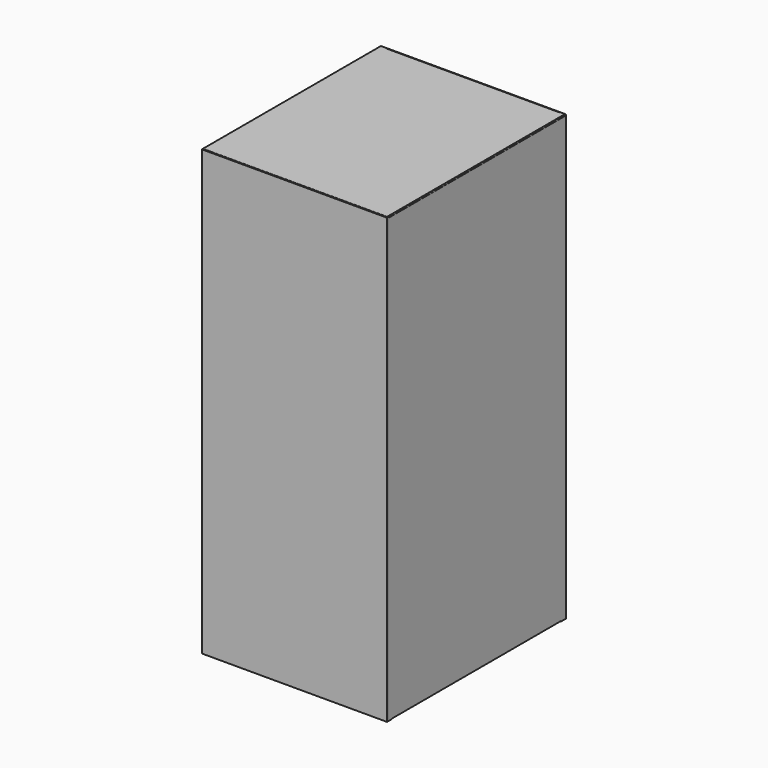
from build123d import *

# Parameters (mm, degrees)
F1_DEPTH       = 914.4
F3_DEPTH       = 1828.8
F5_DEPTH       = 749.3
F6_R           = 6.35
F6_W           = 3.175
F6_H           = 487.3625
F6_H_2         = 6.35
F6_H_3         = 31.75
F7_DEPTH       = 50.8
F7_DEPTH_BACK  = 50.8
F8_W           = 850.9
F8_H           = 1111.25
F9_DEPTH       = 1.016
F10_W          = 3.175
F10_H          = 25.4
F11_DEPTH      = 581.026
F11_DEPTH_BACK = 180.976
F13_W          = 850.9
F13_H          = 1111.25
F14_DEPTH      = 1.016
F12_W          = 914.4
F12_H          = 1823.2365249493
F16_DEPTH      = 0.8128
F15_W          = 920.75
F15_H          = 1828.8
F17_DEPTH      = 0.8128
F18_W          = 758.825
F18_H          = 914.4
F19_DEPTH      = 0.8128
F20_W          = 755.65
F20_H          = 914.4
F21_DEPTH      = 0.8128
F22_W          = 755.65
F22_H          = 1828.8
F23_DEPTH      = 0.8128
F24_W          = 762
F24_H          = 1828.8
F25_DEPTH      = 0.8128


with BuildPart() as f1:
    # F0 (on Front) → F1 (new body)
    with BuildSketch(Plane.XZ):
        Polygon((0, 25.4), (0, 0), (25.4, 0), (25.4, 3.175), (3.175, 3.175), (3.175, 25.4), align=None)
    extrude(amount=-F1_DEPTH)


with BuildPart() as f1b:
    # F0 (on Front) → F1, piece 2 (new body)
    with BuildSketch(Plane.XZ):
        Polygon((730.25, 3.175), (730.25, 0), (755.65, 0), (755.65, 25.4), (752.475, 25.4), (752.475, 3.175), align=None)
    extrude(amount=-F1_DEPTH)


with BuildPart() as f1c:
    # F0 (on Front) → F1, piece 3 (new body)
    with BuildSketch(Plane.XZ):
        Polygon((755.65, 1828.8), (730.25, 1828.8), (730.25, 1825.625), (752.475, 1825.625), (752.475, 1803.4), (755.65, 1803.4), align=None)
    extrude(amount=-F1_DEPTH)


with BuildPart() as f1d:
    # F0 (on Front) → F1, piece 4 (new body)
    with BuildSketch(Plane.XZ):
        Polygon((0, 1828.8), (0, 1803.4), (3.175, 1803.4), (3.175, 1825.625), (25.4, 1825.625), (25.4, 1828.8), align=None)
    extrude(amount=-F1_DEPTH)


with BuildPart() as f1e:
    # F0 (on Front) → F1, piece 5 (new body)
    with BuildSketch(Plane.XZ):
        Polygon((755.65, 635), (717.55, 635), (717.55, 628.65), (749.3, 628.65), (749.3, 596.9), (755.65, 596.9), align=None)
    extrude(amount=-F1_DEPTH)


with BuildPart() as f1f:
    # F0 (on Front) → F1, piece 6 (new body)
    with BuildSketch(Plane.XZ):
        Polygon((0, 635), (0, 596.9), (6.35, 596.9), (6.35, 628.65), (38.1, 628.65), (38.1, 635), align=None)
    extrude(amount=-F1_DEPTH)


with BuildPart() as f1g:
    # F0 (on Front) → F1, piece 7 (new body)
    with BuildSketch(Plane.XZ):
        Polygon((603.25, 736.6), (577.85, 736.6), (577.85, 733.425), (600.075, 733.425), (600.075, 711.2), (603.25, 711.2), align=None)
    extrude(amount=-F1_DEPTH)


with BuildPart() as f1h:
    # F0 (on Front) → F1, piece 8 (new body)
    with BuildSketch(Plane.XZ):
        Polygon((603.25, 1822.45), (577.85, 1822.45), (577.85, 1819.275), (600.075, 1819.275), (600.075, 1797.05), (603.25, 1797.05), align=None)
    extrude(amount=-F1_DEPTH)


with BuildPart() as f1i:
    # F0 (on Front) → F1, piece 9 (new body)
    with BuildSketch(Plane.XZ):
        Polygon((330.2, 733.425), (330.2, 736.6), (304.8, 736.6), (304.8, 711.2), (307.975, 711.2), (307.975, 733.425), align=None)
    extrude(amount=-F1_DEPTH)


with BuildPart() as f1j:
    # F0 (on Front) → F1, piece 10 (new body)
    with BuildSketch(Plane.XZ):
        Polygon((330.2, 1819.275), (330.2, 1822.45), (304.8, 1822.45), (304.8, 1797.05), (307.975, 1797.05), (307.975, 1819.275), align=None)
    extrude(amount=-F1_DEPTH)


with BuildPart() as f3:
    # F2 (on Top) → F3 (new body)
    with BuildSketch(Plane.XY):
        Polygon((0, 22.225), (-3.175, 22.225), (-3.175, -3.175), (22.225, -3.175), (22.225, 0), (0, 0), align=None)
    extrude(amount=F3_DEPTH)


with BuildPart() as f3b:
    # F2 (on Top) → F3, piece 2 (new body)
    with BuildSketch(Plane.XY):
        Polygon((733.425, 0), (733.425, -3.175), (758.825, -3.175), (758.825, 22.225), (755.65, 22.225), (755.65, 0), align=None)
    extrude(amount=F3_DEPTH)


with BuildPart() as f3c:
    # F2 (on Top) → F3, piece 3 (new body)
    with BuildSketch(Plane.XY):
        Polygon((-3.175, 892.175), (0, 892.175), (0, 914.4), (22.225, 914.4), (22.225, 917.575), (-3.175, 917.575), align=None)
    extrude(amount=F3_DEPTH)


with BuildPart() as f3d:
    # F2 (on Top) → F3, piece 4 (new body)
    with BuildSketch(Plane.XY):
        Polygon((733.425, 917.575), (733.425, 914.4), (755.65, 914.4), (755.65, 892.175), (758.825, 892.175), (758.825, 917.575), align=None)
    extrude(amount=F3_DEPTH)


with BuildPart() as f5:
    # F4 (on face) → F5 (new body, through all)
    with BuildSketch(Plane(origin=(752.475, 0, 0), x_dir=(0, -1, 0), z_dir=(-1, 0, 0))):
        Polygon((-25.4, 6.35), (-25.4, 3.175), (0, 3.175), (0, 28.575), (-3.175, 28.575), (-3.175, 6.35), align=None)
    extrude(amount=F5_DEPTH)


with BuildPart() as f5b:
    # F4 (on face) → F5, piece 2 (new body, through all)
    with BuildSketch(Plane(origin=(752.475, 0, 0), x_dir=(0, -1, 0), z_dir=(-1, 0, 0))):
        Polygon((-3.175, 1800.225), (0, 1800.225), (0, 1825.625), (-25.4, 1825.625), (-25.4, 1822.45), (-3.175, 1822.45), align=None)
    extrude(amount=F5_DEPTH)


with BuildPart() as f5c:
    # F4 (on face) → F5, piece 3 (new body, through all)
    with BuildSketch(Plane(origin=(752.475, 0, 0), x_dir=(0, -1, 0), z_dir=(-1, 0, 0))):
        Polygon((-914.4, 1825.625), (-914.4, 1800.225), (-911.225, 1800.225), (-911.225, 1822.45), (-889, 1822.45), (-889, 1825.625), align=None)
    extrude(amount=F5_DEPTH)


with BuildPart() as f5d:
    # F4 (on face) → F5, piece 4 (new body, through all)
    with BuildSketch(Plane(origin=(752.475, 0, 0), x_dir=(0, -1, 0), z_dir=(-1, 0, 0))):
        Polygon((-911.225, 28.575), (-914.4, 28.575), (-914.4, 3.175), (-889, 3.175), (-889, 6.35), (-911.225, 6.35), align=None)
    extrude(amount=F5_DEPTH)


with BuildPart() as f5e:
    # F4 (on face) → F5, piece 5 (new body, through all)
    with BuildSketch(Plane(origin=(752.475, 0, 0), x_dir=(0, -1, 0), z_dir=(-1, 0, 0))):
        Polygon((-573.0875, 628.65), (-573.0875, 590.55), (-566.7375, 590.55), (-566.7375, 622.3), (-534.9875, 622.3), (-534.9875, 628.65), align=None)
    extrude(amount=F5_DEPTH)


with BuildPart() as f5f:
    # F4 (on face) → F5, piece 6 (new body, through all)
    with BuildSketch(Plane(origin=(752.475, 0, 0), x_dir=(0, -1, 0), z_dir=(-1, 0, 0))):
        Polygon((-53.975, 590.55), (-47.625, 590.55), (-47.625, 628.65), (-85.725, 628.65), (-85.725, 622.3), (-53.975, 622.3), align=None)
    extrude(amount=F5_DEPTH)


with BuildPart() as f5g:
    # F4 (on face) → F5, piece 7 (new body, through all)
    with BuildSketch(Plane(origin=(752.475, 0, 0), x_dir=(0, -1, 0), z_dir=(-1, 0, 0))):
        Polygon((-25.4, 736.6), (0, 736.6), (0, 762), (-3.175, 762), (-3.175, 739.775), (-25.4, 739.775), align=None)
    extrude(amount=F5_DEPTH)


with BuildPart() as f5h:
    # F4 (on face) → F5, piece 8 (new body, through all)
    with BuildSketch(Plane(origin=(752.475, 0, 0), x_dir=(0, -1, 0), z_dir=(-1, 0, 0))):
        Polygon((-914.4, 736.6), (-889, 736.6), (-889, 739.775), (-911.225, 739.775), (-911.225, 762), (-914.4, 762), align=None)
    extrude(amount=F5_DEPTH)


with BuildPart() as f7_tool:
    # F6 (on face) → F7 (new body, two sides)
    with BuildSketch(Plane(origin=(0, 0, 622.3), x_dir=(1, 0, 0), z_dir=(0, 0, -1))) as f7_sk:
        with Locations((473.075, -69.85)):
            Circle(F6_R)
        with Locations((473.075, -550.8625)):
            Circle(F6_R)
        with Locations((127, -550.8625)):
            Circle(F6_R)
        with Locations((127, -69.85)):
            Circle(F6_R)
        with Locations((4.7625, -291.30625)):
            Rectangle(F6_W, F6_H)
        with Locations((750.8875, -291.30625)):
            Rectangle(F6_W, F6_H)
        with Locations((4.7625, -569.9125)):
            Rectangle(F6_W, F6_H_2)
        with Locations((4.7625, -550.8625)):
            Rectangle(F6_W, F6_H_3)
        with Locations((750.8875, -550.8625)):
            Rectangle(F6_W, F6_H_3)
        with Locations((750.8875, -569.9125)):
            Rectangle(F6_W, F6_H_2)
    extrude(amount=-F7_DEPTH)
    extrude(f7_sk.sketch, amount=F7_DEPTH_BACK)


with BuildPart() as f5e_1:
    add(f5e.part)

    # F7: cut by f7_tool
    add(f7_tool.part, mode=Mode.SUBTRACT)


with BuildPart() as f5f_1:
    add(f5f.part)

    # F7: cut by f7_tool
    add(f7_tool.part, mode=Mode.SUBTRACT)


with BuildPart() as f9:
    # F8 (on face) → F9 (new body)
    with BuildSketch(Plane.YZ.offset(603.25)):
        with Locations((457.2, 1266.825)):
            Rectangle(F8_W, F8_H)
    extrude(amount=F9_DEPTH)


with BuildPart() as f11_tool:
    # F10 (on face) → F11 (new body, two sides)
    with BuildSketch(Plane(origin=(577.85, 0, 0), x_dir=(0, -1, 0), z_dir=(-1, 0, 0))) as f11_sk:
        with Locations((-1.5875, 1809.75)):
            Rectangle(F10_W, F10_H)
        with Locations((-912.8125, 1809.75)):
            Rectangle(F10_W, F10_H)
    extrude(amount=F11_DEPTH)
    extrude(f11_sk.sketch, amount=-F11_DEPTH_BACK)


with BuildPart() as f1h_1:
    add(f1h.part)

    # F11: cut by f11_tool
    add(f11_tool.part, mode=Mode.SUBTRACT)


with BuildPart() as f1j_1:
    add(f1j.part)

    # F11: cut by f11_tool
    add(f11_tool.part, mode=Mode.SUBTRACT)


with BuildPart() as f14:
    # F13 (on face) → F14 (new body)
    with BuildSketch(Plane(origin=(304.8, 0, 0), x_dir=(0, -1, 0), z_dir=(-1, 0, 0))):
        with Locations((-457.2, 1266.825)):
            Rectangle(F13_W, F13_H)
    extrude(amount=F14_DEPTH)


with BuildPart() as f16:
    # F12 (on face) → F16 (new body)
    with BuildSketch(Plane.YZ.offset(758.825)):
        with Locations((457.2, 914.4)):
            Rectangle(F12_W, F12_H)
    extrude(amount=F16_DEPTH)


with BuildPart() as f17:
    # F15 (on face) → F17 (new body)
    with BuildSketch(Plane(origin=(-3.175, 0, 0), x_dir=(0, -1, 0), z_dir=(-1, 0, 0))):
        with Locations((-457.2, 914.4)):
            Rectangle(F15_W, F15_H)
    extrude(amount=F17_DEPTH)


with BuildPart() as f19:
    # F18 (on face) → F19 (new body)
    with BuildSketch(Plane.XY.offset(1828.8)):
        with Locations((376.2375, 457.2)):
            Rectangle(F18_W, F18_H)
    extrude(amount=F19_DEPTH)


with BuildPart() as f21:
    # F20 (on face) → F21 (new body)
    with BuildSketch(Plane(origin=(0, 0, 0), x_dir=(1, 0, 0), z_dir=(0, 0, -1))):
        with Locations((377.825, -457.2)):
            Rectangle(F20_W, F20_H)
    extrude(amount=F21_DEPTH)


with BuildPart() as f23:
    # F22 (on face) → F23 (new body)
    with BuildSketch(Plane(origin=(0, 917.575, 0), x_dir=(-1, 0, 0), z_dir=(0, 1, 0))):
        with Locations((-377.825, 914.4)):
            Rectangle(F22_W, F22_H)
    extrude(amount=F23_DEPTH)


with BuildPart() as f25:
    # F24 (on face) → F25 (new body)
    with BuildSketch(Plane.XZ.offset(3.175)):
        with Locations((377.825, 914.4)):
            Rectangle(F24_W, F24_H)
    extrude(amount=F25_DEPTH)


solid = Compound([f1.part, f1b.part, f1c.part, f1d.part, f1e.part, f1f.part, f1g.part, f1i.part, f3.part, f3b.part, f3c.part, f3d.part, f5.part, f5b.part, f5c.part, f5d.part, f5g.part, f5h.part, f5e_1.part, f5f_1.part, f9.part, f1h_1.part, f1j_1.part, f14.part, f16.part, f17.part, f19.part, f21.part, f23.part, f25.part])
